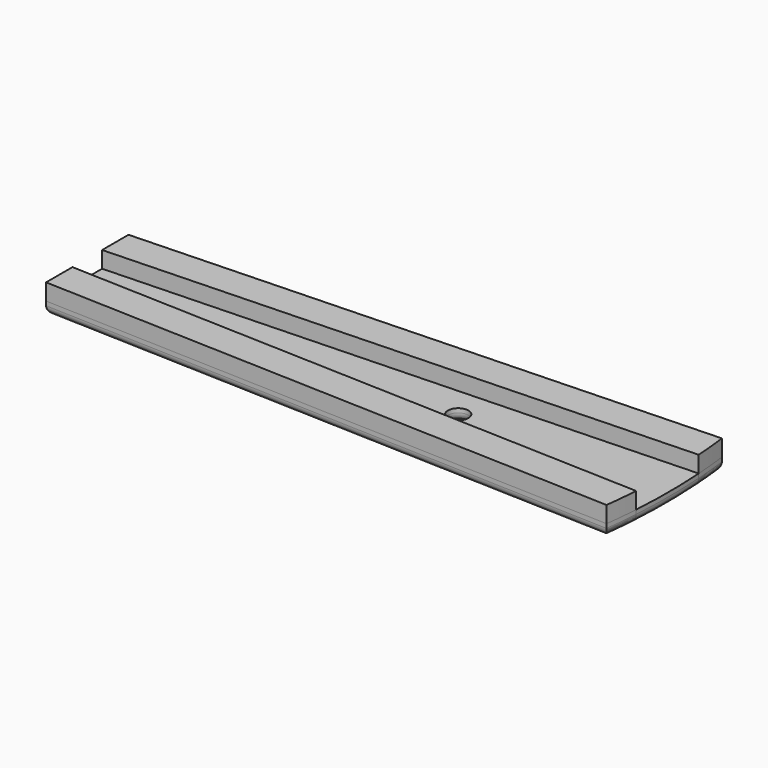
from build123d import *

# Parameters (mm, degrees)
F1_DEPTH = 7
F0_R     = 2.5
F2_DEPTH = 3
F3_R     = 2
F3_2_R   = 2
F3_3_R   = 2


with BuildPart() as f1:
    # F0 (on Top) → F1 (new body)
    with BuildSketch(Plane.XY):
        with BuildLine():
            Line((70, 17.5), (-70, 12.5))
            Line((-70, 12.5), (-70, 4.5))
            Line((-70, 4.5), (70.7693148381, 9.5))
            ThreePointArc((70.7693148381, 9.5), (70.4416321419, 13.5054789375), (70, 17.5))
        make_face()
    extrude(amount=F1_DEPTH)

    # F3#2
    f3_2_edges = [f1.edges().sort_by_distance(p)[0] for p in [
        (0, 15, 0),
        (-70, 8.5, 0),
        (0.384657, 7, 0),
        (70.441632, 13.505479, 0),
    ]]
    fillet(f3_2_edges, radius=F3_2_R)


with BuildPart() as f1b:
    # F0 (on Top) → F1, piece 2 (new body)
    with BuildSketch(Plane.XY):
        with BuildLine():
            Line((70.7693148381, -9.5), (-70, -4.5))
            Line((-70, -4.5), (-70, -12.5))
            Line((-70, -12.5), (70, -17.5))
            ThreePointArc((70, -17.5), (70.4416321419, -13.5054789375), (70.7693148381, -9.5))
        make_face()
    extrude(amount=F1_DEPTH)

    # F3#3
    f3_3_edges = [f1b.edges().sort_by_distance(p)[0] for p in [
        (0, -15, 0),
        (0.384657, -7, 0),
        (-70, -8.5, 0),
        (70.441632, -13.505479, 0),
    ]]
    fillet(f3_3_edges, radius=F3_3_R)


with BuildPart() as f2:
    # F0 (on Top) → F2 (new body)
    with BuildSketch(Plane.XY):
        with BuildLine():
            Line((70, 17.5), (-70, 12.5))
            Line((-70, 12.5), (-70, 4.5))
            Line((-70, 4.5), (70.7693148381, 9.5))
            ThreePointArc((70.7693148381, 9.5), (70.4416321419, 13.5054789375), (70, 17.5))
        make_face()
        with BuildLine():
            Line((70.7693148381, 9.5), (-70, 4.5))
            Line((-70, 4.5), (-70, -4.5))
            Line((-70, -4.5), (70.7693148381, -9.5))
            ThreePointArc((70.7693148381, -9.5), (71.0895105952, 0), (70.7693148381, 9.5))
        make_face()
        with Locations((20, 0)):
            Circle(F0_R, mode=Mode.SUBTRACT)
        with BuildLine():
            Line((70.7693148381, -9.5), (-70, -4.5))
            Line((-70, -4.5), (-70, -12.5))
            Line((-70, -12.5), (70, -17.5))
            ThreePointArc((70, -17.5), (70.4416321419, -13.5054789375), (70.7693148381, -9.5))
        make_face()
    extrude(amount=F2_DEPTH)

    # F3
    f3_edges = [f2.edges().sort_by_distance(p)[0] for p in [
        (0, 15, 0),
        (-70, 0, 0),
        (0, -15, 0),
        (71.089511, 0, 0),
        (17.5, 0, 0),
    ]]
    fillet(f3_edges, radius=F3_R)


solid = Compound([f1.part, f1b.part, f2.part])
